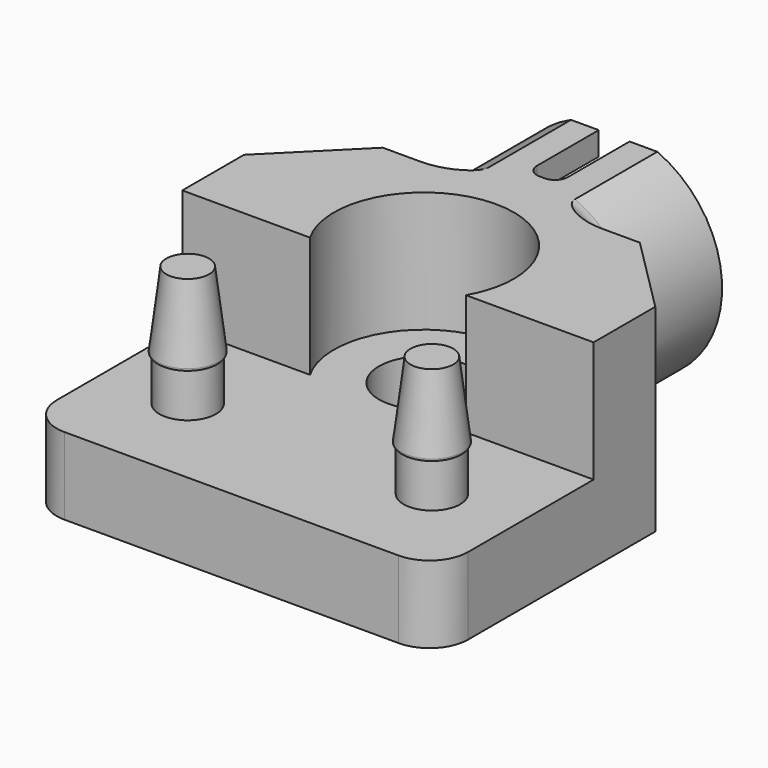
from build123d import *

# Parameters (mm, degrees)
F0_W         = 16
F0_H         = 7.6
F1_DEPTH     = 3
F2_R         = 1.1
F3_DEPTH     = 1.7
F5_R         = 1.2
F6_DEPTH     = 3
F6_TAPER     = 7
F7_S5_R      = 1.1
F7_T6_DEPTH  = 3
F7_S11_R     = 1.1
F7_T12_DEPTH = 3
F4_W         = 16
F4_H         = 6
F8_DEPTH     = 7.7
F9_R         = 3
F10_DEPTH    = 5
F11_W        = 1.2
F11_H        = 3.5
F12_DEPTH    = 7.7
F13_R        = 1.5
F14_R        = 0.5
F16_DEPTH    = 4.7
F17_DEPTH    = 7.7
F18_SIZE     = 3
F19_R        = 1


# Not quite as in the source:
# - a fillet or chamfer that OpenCascade refuses, or shapes differently, is made with other operations: its cross-section is extruded or revolved along the edge and cut away or added


with BuildPart() as f1:
    # F0 (on Top) → F1 (new body)
    with BuildSketch(Plane.XY):
        Rectangle(F0_W, F0_H)
    extrude(amount=F1_DEPTH)

    # F2 (on face) → F3 (join)
    with BuildSketch(Plane.XY.offset(3)):
        with Locations((-4.75, 0)):
            Circle(F2_R)
        with Locations((4.75, 0)):
            Circle(F2_R)
    extrude(amount=F3_DEPTH)

    # F5 (on face) → F6 (join)
    with BuildSketch(Plane.XY.offset(4.7)):
        with Locations((-4.75, 0)):
            Circle(F5_R)
        with Locations((4.75, 0)):
            Circle(F5_R)
    extrude(amount=F6_DEPTH, taper=F6_TAPER)

    # F7: fillet of radius 0.1 on 2 edges, made by hand


with BuildPart() as f7_tool2:
    # F7_s3 → F7_t4 (revolve)
    with BuildSketch(Plane.XZ):
        with BuildLine():
            ThreePointArc((-3.6630294386, 4.7), (-3.5881338666, 4.7337379952), (-3.5637748235, 4.8121869343))
            Line((-3.5637748235, 4.8121869343), (-3.55, 4.7))
            Line((-3.55, 4.7), (-3.6630294386, 4.7))
        make_face()
    revolve(axis=Axis((-4.75, 0, 4.7), (0, 0, -1)))

    # F7_s5 → F7_t6 (cut, symmetric)
    with BuildSketch(Plane.XY.offset(4.8)):
        with Locations((-4.75, 0)):
            Circle(F7_S5_R)
    extrude(amount=F7_T6_DEPTH, both=True, mode=Mode.SUBTRACT)


with BuildPart() as f1_1:
    add(f1.part)

    # F7_t1: cut F7_tool2
    add(f7_tool2.part, mode=Mode.SUBTRACT)


with BuildPart() as f7_tool8:
    # F7_s9 → F7_t10 (revolve)
    with BuildSketch(Plane.XZ):
        with BuildLine():
            ThreePointArc((5.8369705614, 4.7), (5.9118661334, 4.7337379952), (5.9362251765, 4.8121869343))
            Line((5.9362251765, 4.8121869343), (5.95, 4.7))
            Line((5.95, 4.7), (5.8369705614, 4.7))
        make_face()
    revolve(axis=Axis((4.75, 0, 4.7), (0, 0, -1)))

    # F7_s11 → F7_t12 (cut, symmetric)
    with BuildSketch(Plane.XY.offset(4.8)):
        with Locations((4.75, 0)):
            Circle(F7_S11_R)
    extrude(amount=F7_T12_DEPTH, both=True, mode=Mode.SUBTRACT)


with BuildPart() as f1_2:
    add(f1_1.part)

    # F7_t7: cut F7_tool8
    add(f7_tool8.part, mode=Mode.SUBTRACT)

    # F4 (on Top) → F8 (join, through all)
    with BuildSketch(Plane.XY):
        with Locations((0, 6.8)):
            Rectangle(F4_W, F4_H)
    extrude(amount=F8_DEPTH)

    # F9 (on face) → F10 (join)
    with BuildSketch(Plane(origin=(0, 9.8, 0), x_dir=(-1, 0, 0), z_dir=(0, 1, 0))):
        with BuildLine():
            ThreePointArc((1.6785410332, 0), (3.5135361347, 1.5488994306), (4.2, 3.85))
            ThreePointArc((4.2, 3.85), (3.5135361347, 6.1511005694), (1.6785410332, 7.7))
            Line((1.6785410332, 7.7), (-1.6785410332, 7.7))
            ThreePointArc((-1.6785410332, 7.7), (-4.2, 3.85), (-1.6785410332, 0))
            Line((-1.6785410332, 0), (1.6785410332, 0))
        make_face()
        with Locations((0, 3.85)):
            Circle(F9_R, mode=Mode.SUBTRACT)
    extrude(amount=F10_DEPTH)

    # F11 (on face) → F12 (cut, through all)
    with BuildSketch(Plane.XY.offset(7.7)):
        with Locations((0, 13.05)):
            Rectangle(F11_W, F11_H)
    extrude(amount=-F12_DEPTH, mode=Mode.SUBTRACT)

    # F13
    f13_edges = [f1_2.edges().sort_by_distance(p)[0] for p in [
        (-8, -3.8, 1.5),
        (8, -3.8, 1.5),
    ]]
    fillet(f13_edges, radius=F13_R)

    # F14
    f14_edges = [f1_2.edges().sort_by_distance(p)[0] for p in [
        (-0.6, 11.3, 7.244694),
        (0.6, 11.3, 7.244694),
        (0.6, 11.3, 0.455306),
        (-0.6, 11.3, 0.455306),
    ]]
    fillet(f14_edges, radius=F14_R)

    # F15 (on face) → F16 (cut, through all)
    with BuildSketch(Plane.XY.offset(7.7)):
        with BuildLine():
            ThreePointArc((3.0310889132, 3.8), (3.380740392, 4.6441333421), (3.5, 5.55))
            ThreePointArc((3.5, 5.55), (-0.9058666579, 8.930740392), (-3.0310889132, 3.8))
            Line((-3.0310889132, 3.8), (0, 3.8))
            Line((0, 3.8), (3.0310889132, 3.8))
        make_face()
        with BuildLine():
            ThreePointArc((1.75, 5.55), (1.2374368671, 4.3125631329), (0, 3.8))
            ThreePointArc((0, 3.8), (-1.2374368671, 6.7874368671), (1.75, 5.55))
        make_face(mode=Mode.SUBTRACT)
        with BuildLine():
            ThreePointArc((1.75, 5.55), (-1.2374368671, 6.7874368671), (0, 3.8))
            ThreePointArc((0, 3.8), (1.2374368671, 4.3125631329), (1.75, 5.55))
        make_face()
    extrude(amount=-F16_DEPTH, mode=Mode.SUBTRACT)

    # F15 (on face) → F17 (cut, through all)
    with BuildSketch(Plane.XY.offset(7.7)):
        with BuildLine():
            ThreePointArc((1.75, 5.55), (-1.2374368671, 6.7874368671), (0, 3.8))
            ThreePointArc((0, 3.8), (1.2374368671, 4.3125631329), (1.75, 5.55))
        make_face()
    extrude(amount=-F17_DEPTH, mode=Mode.SUBTRACT)

    # F18
    f18_edges = [f1_2.edges().sort_by_distance(p)[0] for p in [
        (-8, 9.8, 3.85),
        (8, 9.8, 3.85),
    ]]
    chamfer(f18_edges, length=F18_SIZE)

    # F19
    f19_edges = [f1_2.edges().sort_by_distance(p)[0] for p in [
        (-4.2, 9.8, 3.85),
        (4.2, 9.8, 3.85),
    ]]
    fillet(f19_edges, radius=F19_R)


solid = f1_2.part
